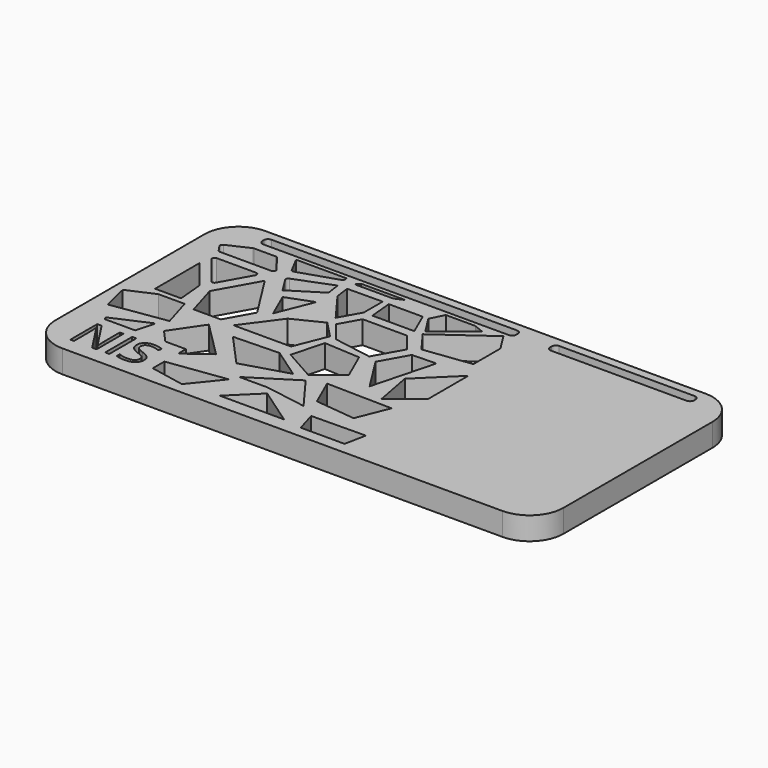
from build123d import *

# Parameters (mm, degrees)
F2_DEPTH     = 27
F1_W         = 4.8709958792
F1_H         = 40
F1_TEXT_SIZE = 55.5555555556
F3_DEPTH     = 27
F5_DEPTH     = 15
F7_DEPTH     = 25


# Not quite as in the source:
# - Text() gives the source's letters only with a copy of the font that has no kerning and outlines rounded to 1/6400 em; it was checked with that copy


with BuildPart() as f2:
    # F0 (on Top) → F2 (new body)
    with BuildSketch(Plane.XY):
        with BuildLine():
            ThreePointArc((300, 110), (288.2842712475, 138.2842712475), (260, 150))
            Line((260, 150), (-260, 150))
            ThreePointArc((-260, 150), (-288.2842712475, 138.2842712475), (-300, 110))
            Line((-300, 110), (-300, -110))
            ThreePointArc((-300, -110), (-288.2842712475, -138.2842712475), (-260, -150))
            Line((-260, -150), (260, -150))
            ThreePointArc((260, -150), (288.2842712475, -138.2842712475), (300, -110))
            Line((300, -110), (300, 110))
        make_face()
    extrude(amount=F2_DEPTH)

    # F1 (on face) → F3 (cut)
    with BuildSketch(Plane.XY):
        with BuildLine():
            Line((-247.795599054, 116.0829370972), (-273.194096087, 104.3470862791))
            ThreePointArc((-273.194096087, 104.3470862791), (-274.8268858979, 102.424522842), (-274.4158693996, 99.935885027))
            Line((-274.4158693996, 99.935885027), (-269.4335967782, 92.6149989031))
            ThreePointArc((-269.4335967782, 92.6149989031), (-268.3563808304, 91.6511158327), (-266.953458595, 91.3028717041))
            Line((-266.953458595, 91.3028717041), (-206.0867457074, 91.3028717041))
            ThreePointArc((-206.0867457074, 91.3028717041), (-203.387751421, 92.9931275146), (-203.730084318, 96.1592518095))
            Line((-203.730084318, 96.1592518095), (-218.7413827133, 115.2159887515))
            ThreePointArc((-218.7413827133, 115.2159887515), (-219.7882999132, 116.0586029325), (-221.0980441027, 116.3596086461))
            Line((-221.0980441027, 116.3596086461), (-246.5372341835, 116.3596086461))
            ThreePointArc((-246.5372341835, 116.3596086461), (-247.1814448038, 116.2896244612), (-247.795599054, 116.0829370972))
        make_face()
        with BuildLine():
            ThreePointArc((-183.5041473559, 89.6143023114), (-185.261412438, 87.7618743164), (-184.9554760756, 85.2269437477))
            Line((-184.9554760756, 85.2269437477), (-173.8530248404, 67.5057247281))
            Line((-173.8530248404, 67.5057247281), (-137.6261113817, 90.2021058085))
            Line((-137.6261113817, 90.2021058085), (-140.0360316038, 106.5831407905))
            Line((-140.0360316038, 106.5831407905), (-183.5041473559, 89.6143023114))
        make_face()
        with BuildLine():
            Line((-142.7033432719, 122.973524034), (-202.2116087957, 122.973524034))
            Line((-202.2116087957, 122.973524034), (-192.5088466294, 104.4776289148))
            ThreePointArc((-192.5088466294, 104.4776289148), (-190.9832826548, 103.0926686401), (-188.9241691005, 103.0184273219))
            Line((-188.9241691005, 103.0184273219), (-144.3617731691, 117.5146339897))
            ThreePointArc((-144.3617731691, 117.5146339897), (-142.7179329636, 118.822991797), (-142.3354580893, 120.8888387767))
            Line((-142.3354580893, 120.8888387767), (-142.7033432719, 122.973524034))
        make_face()
        Polygon((-87.5495970249, 107.4791327119), (-129.2565912008, 107.0578470826), (-126.9395500422, 89.9958983064), (-101.2412905693, 55.2400574088), (-87.5495970249, 79.6744674444), align=None)
        Polygon((-39.9482473731, 107.0578470826), (-79.9790918827, 107.0578470826), (-77.4993076921, 79.6744674444), (-27.9035717249, 79.6744674444), align=None)
        with BuildLine():
            ThreePointArc((-261.3570791085, 79.6744674444), (-264.0591763899, 77.9777979021), (-263.7048962327, 74.806914299))
            Line((-263.7048962327, 74.806914299), (-236.398176882, 40.477940339))
            ThreePointArc((-236.398176882, 40.477940339), (-233.8088140593, 39.3552333493), (-231.4332264479, 40.8789965569))
            Line((-231.4332264479, 40.8789965569), (-212.1971658895, 75.2079705169))
            ThreePointArc((-212.1971658895, 75.2079705169), (-212.2259125607, 78.1911264729), (-214.8142991994, 79.6744674444))
            Line((-214.8142991994, 79.6744674444), (-261.3570791085, 79.6744674444))
        make_face()
        Polygon((-164.2758161113, 18.0218300183), (-198.5099166632, 72.1014514565), (-225.3133413571, 24.2676413288), (-214.0406817198, -13.5682784021), (-181.9771677256, -13.5682784021), align=None)
        Polygon((-134.8269730806, 68.4951916337), (-165.3875261545, 56.9723658264), (-151.8282156103, 26.1454877013), align=None)
        Polygon((-239.6457042439, 27.1545214449), (-267.5767540932, 62.2683800757), (-267.5767540932, -3.5485028363), (-236.8652996618, -3.5485028363), align=None)
        Polygon((-101.2412905693, 42.7296645939), (-134.8269730806, 26.196911931), (-165.3875261545, -15.3854712844), (-97.5513607264, -15.3854712844), (-82.1636760065, 22.9448972727), align=None)
        Polygon((-125.4195418774, 122.973524034), (-129.2565912008, 118.3211952448), (-83.9025080204, 118.3211952448), (-73.3255120798, 122.973524034), align=None)
        Polygon((-25.3802469761, 122.973524034), (-33.2954898477, 107.0578470826), (-19.8547632255, 85.8255262135), (20.9975618619, 118.3211952448), (9.4087179009, 122.973524034), align=None)
        Polygon((42.6593485126, 122.973524034), (42.5151288509, 123.2013478875), (42.1980379991, 122.973524034), align=None)
        Polygon((55.7874693389, 102.2350266576), (42.6593485126, 122.973524034), (42.1980379991, 122.973524034), (-18.0666556454, 79.6744674444), (0, 55.2400574088), (55.7874693389, 62.2683800757), align=None)
        Polygon((-27.344670818, 68.4951916337), (-79.9790918827, 68.4951916337), (-92.8574785679, 45.5122217152), (-73.9883727745, 21.7906961407), (-28.8295261562, 14.1261443496), (-10.3417352429, 47.11974462), align=None)
        Polygon((-35.0691898255, 7.0528669597), (-77.4993076921, 9.5774251968), (-87.5495970249, -28.4980107099), (-49.324458652, -49.9172665679), (-20.2005089569, -26.7508438943), align=None)
        Polygon((28.3302999133, 41.9490246602), (0, 41.1399565637), (-17.6858989569, 9.5774251968), (8.7588300205, -32.1973230538), align=None)
        Polygon((66.6768550873, 41.1399565637), (24.5934743434, 0), (33.0009584069, -44.7644009526), (66.6768550873, -17.9771669209), align=None)
        Polygon((-258.2386194972, -10.0816944138), (-289.5357608795, -23.8478519022), (-282.0208668709, -55.4103851318), (-216.8374396425, -45.5767928027), (-227.4126857519, -10.0816944138), align=None)
        Polygon((-141.8823450804, -70.6341216725), (-184.0637177229, -28.4980107099), (-208.4908485413, -64.2739385366), (-194.3093136996, -80), (-170, -80), (-170, -91.424146406), align=None)
        Polygon((-97.667984551, -32.0510392469), (-151.5934914351, -33.5910655558), (-116.0154960522, -72.9412159263), (-61.928011477, -56.8266399205), align=None)
        Polygon((51.9334782601, -53.8158046363), (-25.2873059362, -52.3582585156), (-10.5282225491, -85.9128012286), (36.972116679, -91.0842120647), align=None)
        Polygon((-223.8779127827, -57.4363257051), (-267.5767540932, -76.6574144363), (-265.9785781204, -80), (-229.8337593719, -80), align=None)
        Polygon((-170, -111.7559216835), (-170, -128.8925153788), (-129.2565912008, -136.900857091), (-101.2412905693, -102.3556664586), align=None)
        Polygon((-96.7199504375, -92.66615659), (-63.4386092424, -92.66615659), (-14.3575508386, -100.8429764941), (-44.7353399723, -59.758263848), align=None)
        Polygon((-56.0946115553, -102.2792782824), (-87.5495970249, -133.1093162298), (-11.6208270192, -133.1093162298), align=None)
        Polygon((67.4672139422, -111.1876231625), (3.5453645978, -112.0451688766), (10.7812651266, -136.3319796556), (62.5249519944, -136.3319796556), align=None)
        with Locations((-221.5732261539, -111.7405728251)):
            Rectangle(F1_W, F1_H)
        with Locations((-270.518168807, -131.7405728251)):
            Text('N S', F1_TEXT_SIZE, font='Open Sans', text_align=(TextAlign.LEFT, TextAlign.BOTTOM))
    extrude(amount=F3_DEPTH, mode=Mode.SUBTRACT)

    # F4 (on face) → F5 (cut)
    with BuildSketch(Plane.XY.offset(27)):
        with BuildLine():
            Line((45, 140), (-245, 140))
            ThreePointArc((-245, 140), (-248.5355339059, 138.5355339059), (-250, 135))
            Line((-250, 135), (-250, 133))
            ThreePointArc((-250, 133), (-248.5355339059, 129.4644660941), (-245, 128))
            Line((-245, 128), (45, 128))
            ThreePointArc((45, 128), (48.5355339059, 129.4644660941), (50, 133))
            Line((50, 133), (50, 135))
            ThreePointArc((50, 135), (48.5355339059, 138.5355339059), (45, 140))
        make_face()
        with BuildLine():
            Line((255, 140), (95, 140))
            ThreePointArc((95, 140), (91.4644660941, 138.5355339059), (90, 135))
            Line((90, 135), (90, 133))
            ThreePointArc((90, 133), (91.4644660941, 129.4644660941), (95, 128))
            Line((95, 128), (255, 128))
            ThreePointArc((255, 128), (258.5355339059, 129.4644660941), (260, 133))
            Line((260, 133), (260, 135))
            ThreePointArc((260, 135), (258.5355339059, 138.5355339059), (255, 140))
        make_face()
    extrude(amount=-F5_DEPTH, mode=Mode.SUBTRACT)

    # F6 (on face) → F7 (cut)
    with BuildSketch(Plane.XY.offset(12)):
        with BuildLine():
            Line((-106, 130), (-94, 130))
            ThreePointArc((-94, 130), (-91.1715728753, 131.1715728753), (-90, 134))
            ThreePointArc((-90, 134), (-91.1715728753, 136.8284271247), (-94, 138))
            Line((-94, 138), (-106, 138))
            ThreePointArc((-106, 138), (-108.8284271247, 136.8284271247), (-110, 134))
            ThreePointArc((-110, 134), (-108.8284271247, 131.1715728753), (-106, 130))
        make_face()
        with BuildLine():
            Line((169, 130), (181, 130))
            ThreePointArc((181, 130), (183.8284271247, 131.1715728753), (185, 134))
            ThreePointArc((185, 134), (183.8284271247, 136.8284271247), (181, 138))
            Line((181, 138), (169, 138))
            ThreePointArc((169, 138), (166.1715728753, 136.8284271247), (165, 134))
            ThreePointArc((165, 134), (166.1715728753, 131.1715728753), (169, 130))
        make_face()
    extrude(amount=-F7_DEPTH, mode=Mode.SUBTRACT)


solid = f2.part
